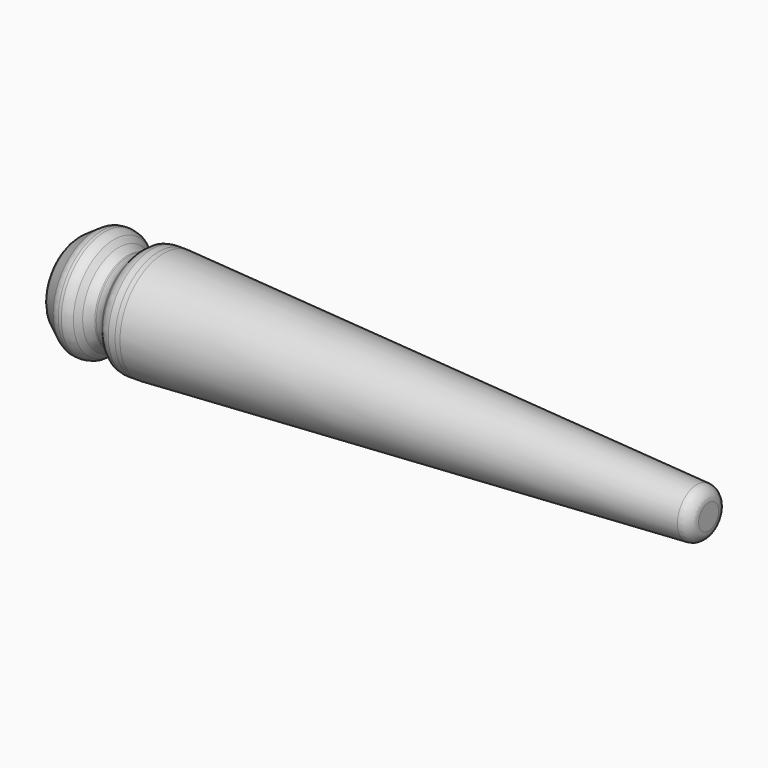
from build123d import *

# Parameters (mm, degrees)
F0_R       = 2.25
F1_DEPTH   = 0.5
F3_START   = 1
F2_R       = 1.7
F3_DEPTH   = 0.5
F1_FACE_R  = 2.25
F3_FACE_R  = 1.7
F6_START   = 2
F5_R       = 2.25
F6_DEPTH   = 0.5
F6_FACE_R  = 2.25
F3_FACE1_R = 1.7
F8_R       = 0.5
F10_START  = -0.8
F9_R       = 1.7
F10_DEPTH  = 0.2
F10_FACE_R = 1.7
F1_FACE1_R = 2.25
F13_R      = 0.5
F15_START  = 2.5
F14_R      = 2.25
F15_DEPTH  = 0.2
F17_START  = 25
F16_R      = 1
F17_DEPTH  = 0.2
F15_FACE_R = 2.25
F17_FACE_R = 1
F19_R      = 0.5


# Not quite as in the source:
# - a fillet or chamfer that OpenCascade refuses, or shapes differently, is made with other operations: its cross-section is extruded or revolved along the edge and cut away or added


with BuildPart() as f1:
    # F0 (on Right) → F1 (new body)
    with BuildSketch(Plane.YZ):
        Circle(F0_R)
    extrude(amount=F1_DEPTH)



with BuildPart() as f3:
    # F2 (on Right) → F3 (new body)
    with BuildSketch(Plane.YZ.offset(F3_START)):
        Circle(F2_R)
    extrude(amount=F3_DEPTH)


with BuildPart() as f1_1:
    add(f1.part)

    add(f3.part)  # F4 merges F3
    # F1_face (on face) → F4 section 0
    with BuildSketch(Plane.YZ.offset(0.5)):
        Circle(F1_FACE_R)
    # F3_face (on face) → F4 section 1
    with BuildSketch(Plane(origin=(1, 0, 0), x_dir=(0, 1, 0), z_dir=(-1, 0, 0))):
        Circle(F3_FACE_R)
    loft()



with BuildPart() as f6:
    # F5 (on Right) → F6 (new body)
    with BuildSketch(Plane.YZ.offset(F6_START)):
        Circle(F5_R)
    extrude(amount=F6_DEPTH)


with BuildPart() as f1_2:
    add(f1_1.part)

    add(f6.part)  # F7 merges F6
    # F6_face (on face) → F7 section 0
    with BuildSketch(Plane(origin=(2, 0, 0), x_dir=(0, 1, 0), z_dir=(-1, 0, 0))):
        Circle(F6_FACE_R)
    # F3_face1 (on face) → F7 section 1
    with BuildSketch(Plane.YZ.offset(1.5)):
        Circle(F3_FACE1_R)
    loft()

    # F8
    f8_edges = [f1_2.edges().sort_by_distance(p)[0] for p in [
        (0.5, -2.25, 0),
        (0.75, 1.975, 0),
        (1, -1.7, 0),
        (2, -2.25, 0),
        (1.75, 1.975, 0),
        (1.5, -1.7, 0),
    ]]
    fillet(f8_edges, radius=F8_R)



with BuildPart() as f10:
    # F9 (on Right) → F10 (new body)
    with BuildSketch(Plane.YZ.offset(F10_START)):
        Circle(F9_R)
    extrude(amount=-F10_DEPTH)


with BuildPart() as f1_3:
    add(f1_2.part)

    add(f10.part)  # F11 merges F10
    # F10_face (on face) → F11 section 0
    with BuildSketch(Plane.YZ.offset(-0.8)):
        Circle(F10_FACE_R)
    # F1_face1 (on face) → F11 section 1
    with BuildSketch(Plane(origin=(0, 0, 0), x_dir=(0, 1, 0), z_dir=(-1, 0, 0))):
        Circle(F1_FACE1_R)
    loft()

    # F12: fillet of radius 1 on 1 edges, made by hand

    # F12_s1 → F12_t2 (revolve, cut)
    with BuildSketch(Plane.XY):
        with BuildLine():
            ThreePointArc((-0.8, 1.7), (-0.9486832981, 1.416227766), (-1, 1.1))
            Line((-1, 1.1), (-1.02, 1.1))
            Line((-1.02, 1.1), (-1.02, 1.7))
            Line((-1.02, 1.7), (-1, 1.72))
            ThreePointArc((-1, 1.72), (-0.9, 1.72), (-0.816, 1.712))
            Line((-0.816, 1.712), (-0.8, 1.7))
        make_face()
    revolve(axis=Axis((-1, 0, 0), (1, 0, 0)), mode=Mode.SUBTRACT)

    # F13
    f13_edges = [f1_3.edges().sort_by_distance(p)[0] for p in [
        (-0.8, -1.7, 0),
        (-0.4, 1.975, 0),
        (0, -2.25, 0),
    ]]
    fillet(f13_edges, radius=F13_R)


with BuildPart() as f15:
    # F14 (on Right) → F15 (new body)
    with BuildSketch(Plane.YZ.offset(F15_START)):
        Circle(F14_R)
    extrude(amount=F15_DEPTH)



with BuildPart() as f17:
    # F16 (on Right) → F17 (new body)
    with BuildSketch(Plane.YZ.offset(F17_START)):
        Circle(F16_R)
    extrude(amount=F17_DEPTH)


with BuildPart() as f15_1:
    add(f15.part)

    add(f17.part)  # F18 merges F17
    # F15_face (on face) → F18 section 0
    with BuildSketch(Plane.YZ.offset(2.7)):
        Circle(F15_FACE_R)
    # F17_face (on face) → F18 section 1
    with BuildSketch(Plane(origin=(25, 0, 0), x_dir=(0, 1, 0), z_dir=(-1, 0, 0))):
        Circle(F17_FACE_R)
    loft()

    # F19
    f19_edges = [f15_1.edges().sort_by_distance(p)[0] for p in [
        (25.2, -1, 0),
    ]]
    fillet(f19_edges, radius=F19_R)


solid = Compound([f1_3.part, f15_1.part])
